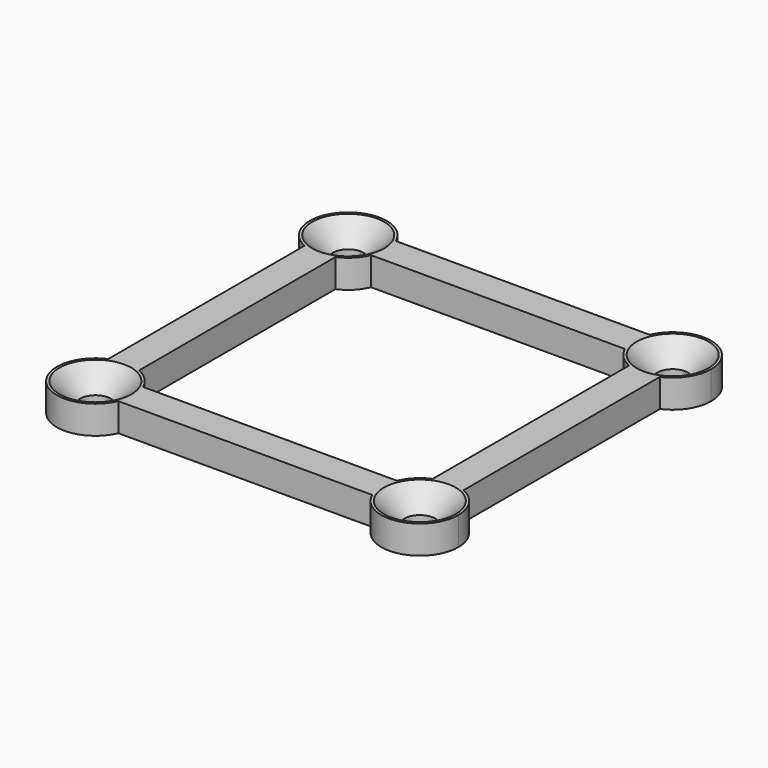
from build123d import *

# Parameters (mm, degrees)
F1_DEPTH = 2.75


# Not quite as in the source:
# - a fillet or chamfer that OpenCascade refuses, or shapes differently, is made with other operations: its cross-section is extruded or revolved along the edge and cut away or added


with BuildPart() as f1:
    # F0 (on Top) → F1 (new body)
    with BuildSketch(Plane.XY):
        with BuildLine():
            ThreePointArc((-15.79, 16.88), (-14.7293398282, 16.4406601718), (-14.29, 15.38))
            Line((-14.29, 15.38), (-14.29, 13.88))
            Line((-14.29, 13.88), (-12.3530682288, 13.88))
            ThreePointArc((-12.3530682288, 13.88), (-12.1191013265, 14.6138388362), (-12.04, 15.38))
            ThreePointArc((-12.04, 15.38), (-12.1191013265, 16.1461611638), (-12.3530682288, 16.88))
            Line((-12.3530682288, 16.88), (-15.79, 16.88))
        make_face()
        with BuildLine():
            ThreePointArc((-17.29, 15.38), (-16.8506601718, 16.4406601718), (-15.79, 16.88))
            Line((-15.79, 16.88), (-12.3530682288, 16.88))
            ThreePointArc((-12.3530682288, 16.88), (-18.4416504294, 18.0316504294), (-17.29, 11.9430682288))
            Line((-17.29, 11.9430682288), (-17.29, 15.38))
        make_face()
        with BuildLine():
            Line((-14.29, 13.88), (-15.79, 13.88))
            ThreePointArc((-15.79, 13.88), (-16.8506601718, 14.3193398282), (-17.29, 15.38))
            Line((-17.29, 15.38), (-17.29, 11.9430682288))
            ThreePointArc((-17.29, 11.9430682288), (-15.79, 11.63), (-14.29, 11.9430682288))
            Line((-14.29, 11.9430682288), (-14.29, 13.88))
        make_face()
        with BuildLine():
            Line((12.3530682288, 16.88), (-12.3530682288, 16.88))
            ThreePointArc((-12.3530682288, 16.88), (-12.1191013265, 16.1461611638), (-12.04, 15.38))
            ThreePointArc((-12.04, 15.38), (-12.1191013265, 14.6138388362), (-12.3530682288, 13.88))
            Line((-12.3530682288, 13.88), (12.3530682288, 13.88))
            ThreePointArc((12.3530682288, 13.88), (12.04, 15.38), (12.3530682288, 16.88))
        make_face()
        with BuildLine():
            Line((-14.29, -11.9430682288), (-14.29, 11.9430682288))
            ThreePointArc((-14.29, 11.9430682288), (-15.79, 11.63), (-17.29, 11.9430682288))
            Line((-17.29, 11.9430682288), (-17.29, -11.9430682288))
            ThreePointArc((-17.29, -11.9430682288), (-15.79, -11.63), (-14.29, -11.9430682288))
        make_face()
        with BuildLine():
            Line((15.79, 16.88), (12.3530682288, 16.88))
            ThreePointArc((12.3530682288, 16.88), (12.04, 15.38), (12.3530682288, 13.88))
            Line((12.3530682288, 13.88), (14.29, 13.88))
            Line((14.29, 13.88), (14.29, 15.38))
            ThreePointArc((14.29, 15.38), (14.7293398282, 16.4406601718), (15.79, 16.88))
        make_face()
        with BuildLine():
            ThreePointArc((19.54, 15.38), (16.5561611638, 19.0508986735), (12.3530682288, 16.88))
            Line((12.3530682288, 16.88), (15.79, 16.88))
            ThreePointArc((15.79, 16.88), (16.8506601718, 16.4406601718), (17.29, 15.38))
            Line((17.29, 15.38), (17.29, 11.9430682288))
            ThreePointArc((17.29, 11.9430682288), (18.9274750995, 13.3260404094), (19.54, 15.38))
        make_face()
        with BuildLine():
            Line((-14.29, -13.88), (-14.29, -11.9430682288))
            ThreePointArc((-14.29, -11.9430682288), (-15.79, -11.63), (-17.29, -11.9430682288))
            Line((-17.29, -11.9430682288), (-17.29, -15.38))
            ThreePointArc((-17.29, -15.38), (-16.8506601718, -14.3193398282), (-15.79, -13.88))
            Line((-15.79, -13.88), (-14.29, -13.88))
        make_face()
        with BuildLine():
            Line((-17.29, -15.38), (-17.29, -11.9430682288))
            ThreePointArc((-17.29, -11.9430682288), (-18.4416504294, -18.0316504294), (-12.3530682288, -16.88))
            Line((-12.3530682288, -16.88), (-15.79, -16.88))
            ThreePointArc((-15.79, -16.88), (-16.8506601718, -16.4406601718), (-17.29, -15.38))
        make_face()
        with BuildLine():
            Line((12.3530682288, -13.88), (-12.3530682288, -13.88))
            ThreePointArc((-12.3530682288, -13.88), (-12.1191013265, -14.6138388362), (-12.04, -15.38))
            ThreePointArc((-12.04, -15.38), (-12.1191013265, -16.1461611638), (-12.3530682288, -16.88))
            Line((-12.3530682288, -16.88), (12.3530682288, -16.88))
            ThreePointArc((12.3530682288, -16.88), (12.04, -15.38), (12.3530682288, -13.88))
        make_face()
        with BuildLine():
            ThreePointArc((-12.04, -15.38), (-12.1191013265, -14.6138388362), (-12.3530682288, -13.88))
            Line((-12.3530682288, -13.88), (-14.29, -13.88))
            Line((-14.29, -13.88), (-14.29, -15.38))
            ThreePointArc((-14.29, -15.38), (-14.7293398282, -16.4406601718), (-15.79, -16.88))
            Line((-15.79, -16.88), (-12.3530682288, -16.88))
            ThreePointArc((-12.3530682288, -16.88), (-12.1191013265, -16.1461611638), (-12.04, -15.38))
        make_face()
        with BuildLine():
            Line((14.29, 13.88), (14.29, 11.9430682288))
            ThreePointArc((14.29, 11.9430682288), (15.79, 11.63), (17.29, 11.9430682288))
            Line((17.29, 11.9430682288), (17.29, 15.38))
            ThreePointArc((17.29, 15.38), (16.8506601718, 14.3193398282), (15.79, 13.88))
            Line((15.79, 13.88), (14.29, 13.88))
        make_face()
        with BuildLine():
            ThreePointArc((17.29, 11.9430682288), (15.79, 11.63), (14.29, 11.9430682288))
            Line((14.29, 11.9430682288), (14.29, -11.9430682288))
            ThreePointArc((14.29, -11.9430682288), (15.79, -11.63), (17.29, -11.9430682288))
            Line((17.29, -11.9430682288), (17.29, 11.9430682288))
        make_face()
        with BuildLine():
            Line((14.29, -13.88), (12.3530682288, -13.88))
            ThreePointArc((12.3530682288, -13.88), (12.04, -15.38), (12.3530682288, -16.88))
            Line((12.3530682288, -16.88), (15.79, -16.88))
            ThreePointArc((15.79, -16.88), (14.7293398282, -16.4406601718), (14.29, -15.38))
            Line((14.29, -15.38), (14.29, -13.88))
        make_face()
        with BuildLine():
            ThreePointArc((17.29, -11.9430682288), (15.79, -11.63), (14.29, -11.9430682288))
            Line((14.29, -11.9430682288), (14.29, -13.88))
            Line((14.29, -13.88), (15.79, -13.88))
            ThreePointArc((15.79, -13.88), (16.8506601718, -14.3193398282), (17.29, -15.38))
            Line((17.29, -15.38), (17.29, -11.9430682288))
        make_face()
        with BuildLine():
            Line((15.79, -16.88), (12.3530682288, -16.88))
            ThreePointArc((12.3530682288, -16.88), (16.5561611638, -19.0508986735), (19.54, -15.38))
            ThreePointArc((19.54, -15.38), (18.9274750995, -13.3260404094), (17.29, -11.9430682288))
            Line((17.29, -11.9430682288), (17.29, -15.38))
            ThreePointArc((17.29, -15.38), (16.8506601718, -16.4406601718), (15.79, -16.88))
        make_face()
        with BuildLine():
            Line((-14.29, 13.88), (-14.29, 15.38))
            ThreePointArc((-14.29, 15.38), (-14.7293398282, 14.3193398282), (-15.79, 13.88))
            Line((-15.79, 13.88), (-14.29, 13.88))
        make_face()
        with BuildLine():
            Line((-12.3530682288, 13.88), (-14.29, 13.88))
            Line((-14.29, 13.88), (-14.29, 11.9430682288))
            ThreePointArc((-14.29, 11.9430682288), (-13.1383495706, 12.7283495706), (-12.3530682288, 13.88))
        make_face()
        with BuildLine():
            Line((14.29, 13.88), (12.3530682288, 13.88))
            ThreePointArc((12.3530682288, 13.88), (13.1383495706, 12.7283495706), (14.29, 11.9430682288))
            Line((14.29, 11.9430682288), (14.29, 13.88))
        make_face()
        with BuildLine():
            Line((14.29, 15.38), (14.29, 13.88))
            Line((14.29, 13.88), (15.79, 13.88))
            ThreePointArc((15.79, 13.88), (14.7293398282, 14.3193398282), (14.29, 15.38))
        make_face()
        with BuildLine():
            Line((-14.29, -15.38), (-14.29, -13.88))
            Line((-14.29, -13.88), (-15.79, -13.88))
            ThreePointArc((-15.79, -13.88), (-14.7293398282, -14.3193398282), (-14.29, -15.38))
        make_face()
        with BuildLine():
            ThreePointArc((-12.3530682288, -13.88), (-13.1383495706, -12.7283495706), (-14.29, -11.9430682288))
            Line((-14.29, -11.9430682288), (-14.29, -13.88))
            Line((-14.29, -13.88), (-12.3530682288, -13.88))
        make_face()
        with BuildLine():
            Line((15.79, -13.88), (14.29, -13.88))
            Line((14.29, -13.88), (14.29, -15.38))
            ThreePointArc((14.29, -15.38), (14.7293398282, -14.3193398282), (15.79, -13.88))
        make_face()
        with BuildLine():
            ThreePointArc((14.29, -11.9430682288), (13.1383495706, -12.7283495706), (12.3530682288, -13.88))
            Line((12.3530682288, -13.88), (14.29, -13.88))
            Line((14.29, -13.88), (14.29, -11.9430682288))
        make_face()
    extrude(amount=F1_DEPTH)

    # F2: chamfer of 2 on 4 edges, made by hand

    # F2_s1 → F2_t2 (revolve, cut)
    with BuildSketch(Plane.XZ.offset(-15.38)):
        Polygon((-14.29, 0.75), (-12.29, 2.75), (-14.29, 2.75), align=None)
    revolve(axis=Axis((-15.79, 15.38, 2.75), (0, 0, -1)), mode=Mode.SUBTRACT)

    # F2_s3 → F2_t4 (revolve, cut)
    with BuildSketch(Plane.YZ.offset(15.79)):
        Polygon((13.88, 0.75), (11.88, 2.75), (13.88, 2.75), align=None)
    revolve(axis=Axis((15.79, 15.38, 2.75), (0, 0, -1)), mode=Mode.SUBTRACT)

    # F2_s5 → F2_t6 (revolve, cut)
    with BuildSketch(Plane.XZ.offset(15.38)):
        Polygon((14.29, 0.75), (12.29, 2.75), (14.29, 2.75), align=None)
    revolve(axis=Axis((15.79, -15.38, 2.75), (0, 0, -1)), mode=Mode.SUBTRACT)

    # F2_s7 → F2_t8 (revolve, cut)
    with BuildSketch(Plane.YZ.offset(-15.79)):
        Polygon((-13.88, 0.75), (-11.88, 2.75), (-13.88, 2.75), align=None)
    revolve(axis=Axis((-15.79, -15.38, 2.75), (0, 0, -1)), mode=Mode.SUBTRACT)


solid = f1.part
